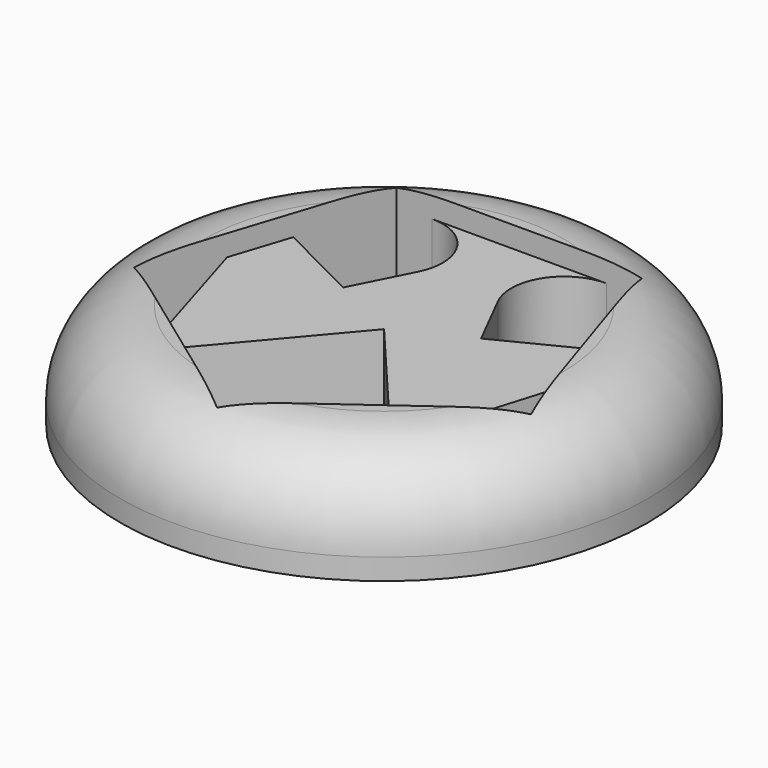
from build123d import *

# Parameters (mm, degrees)
F0_R     = 25
F1_DEPTH = 10
F4_DEPTH = 8
F5_R     = 5


# Not quite as in the source:
# - a fillet or chamfer that OpenCascade refuses, or shapes differently, is made with other operations: its cross-section is extruded or revolved along the edge and cut away or added


with BuildPart() as f1:
    # F0 (on Top) → F1 (new body)
    with BuildSketch(Plane.XY):
        Circle(F0_R)
        Polygon((-18.8114806731, -6.112220586), (-11.6261344347, 16.0020012408), (11.6261344347, 16.0020012408), (18.8114806731, -6.112220586), (0, -19.7795613097), align=None, mode=Mode.SUBTRACT)
    extrude(amount=F1_DEPTH)

    # F2: fillet of radius 8 on 1 edges, made by hand

    # F2_s1 → F2_t2 (revolve, cut)
    with BuildSketch(Plane.XZ):
        with BuildLine():
            ThreePointArc((25, 2), (22.6568542495, 7.6568542495), (17, 10))
            Line((17, 10), (25, 10))
            Line((25, 10), (25, 2))
        make_face()
    revolve(axis=Axis((0, 0, 10), (0, 0, 1)), mode=Mode.SUBTRACT)

    # F3 (on Top) → F4 (join)
    with BuildSketch(Plane.XY):
        Polygon((6.539323839, 3.3114300304), (0, 0), (11.5929096937, -13.7071507052), (18.5771044344, 9.4072083011), align=None)
        Polygon((-6.539323839, 3.3114300304), (0, 0), (6.539323839, 3.3114300304), (0, 16.2251126021), align=None)
        Polygon((-11.5929096937, -13.7071507052), (0, 0), (-6.539323839, 3.3114300304), (-18.5771044344, 9.4072083011), align=None)
    extrude(amount=F4_DEPTH)

    # F5
    f5_edges = [f1.edges().sort_by_distance(p)[0] for p in [
        (-0.112981, 16.002001, 4),
        (0.112981, 16.002001, 4),
    ]]
    fillet(f5_edges, radius=F5_R)


solid = f1.part
